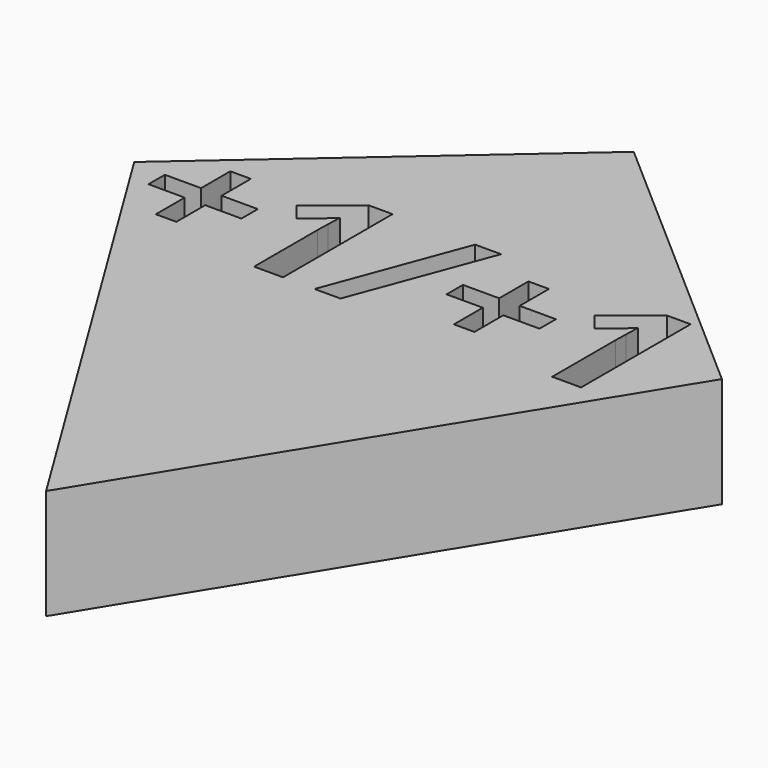
from build123d import *

# Parameters (mm, degrees)
F1_DEPTH     = 3
F2_TEXT_SIZE = 5.2201095968
F3_DEPTH     = 2


# Not quite as in the source:
# - Text() gives the source's letters only with a copy of the font that has no kerning and outlines rounded to 1/6400 em; it was checked with that copy


with BuildPart() as f1:
    # F0 (on Top) → F1 (new body)
    with BuildSketch(Plane.XY):
        Polygon((8, 0), (0, 7), (-8, 0), (0, -13), align=None)
    extrude(amount=F1_DEPTH)

    # F2 (on face) → F3 (cut)
    with BuildSketch(Plane.XY.offset(3)):
        with Locations((-7.3487665504, -2.1705714753)):
            Text('+1/+1', F2_TEXT_SIZE, font='Open Sans', font_style=FontStyle.BOLD, text_align=(TextAlign.LEFT, TextAlign.BOTTOM))
    extrude(amount=-F3_DEPTH, mode=Mode.SUBTRACT)


solid = f1.part
